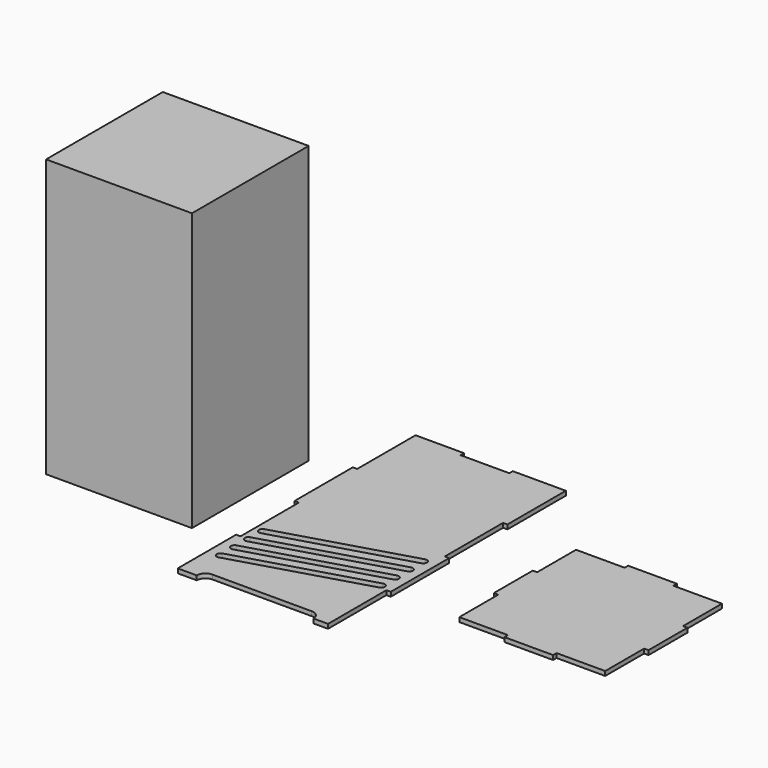
from build123d import *

# Parameters (mm, degrees)
F1_DEPTH = 3
F2_W     = 100
F2_H     = 100
F3_DEPTH = 190


# Not quite as in the source:
# - a feature names something its author has since deleted; it is built from what else it names


with BuildPart() as f1:
    # F0 (on Top) → F1 (new body)
    with BuildSketch(Plane.XY):
        with BuildLine():
            Line((-16.6666666667, 100), (-50, 100))
            Line((-50, 100), (-50, 50))
            Line((-50, 50), (-53, 50))
            Line((-53, 50), (-53, 0))
            Line((-53, 0), (-50, 0))
            Line((-50, 0), (-50, -50))
            Line((-50, -50), (-53, -50))
            Line((-53, -50), (-53, -100))
            Line((-53, -100), (-50, -100))
            Line((-50, -100), (-40, -100))
            ThreePointArc((-40, -100), (-38.2426406871, -95.7573593129), (-34, -94))
            Line((-34, -94), (34, -94))
            ThreePointArc((34, -94), (38.2426406871, -95.7573593129), (40, -100))
            Line((40, -100), (50, -100))
            Line((50, -100), (50, -50))
            Line((50, -50), (53, -50))
            Line((53, -50), (53, 0))
            Line((53, 0), (50, 0))
            Line((50, 0), (50, 50))
            Line((50, 50), (53, 50))
            Line((53, 50), (53, 100))
            Line((53, 100), (50, 100))
            Line((50, 100), (16.6666666667, 100))
            Line((16.6666666667, 100), (16.6666666667, 97))
            Line((16.6666666667, 97), (-16.6666666667, 97))
            Line((-16.6666666667, 97), (-16.6666666667, 100))
        make_face()
        with BuildLine():
            ThreePointArc((-43.7245756516, -76.3485534214), (-46.8767029852, -74.7472747846), (-45.2754243484, -71.595147451))
            Line((-45.2754243484, -71.595147451), (43.7885479556, -45.1109843029))
            ThreePointArc((43.7885479556, -45.1109843029), (46.8963350712, -46.7941332679), (45.2131861062, -49.9019203835))
            Line((45.2131861062, -49.9019203835), (-43.7245756516, -76.3485534214))
        make_face(mode=Mode.SUBTRACT)
        with BuildLine():
            Line((45.2131861062, -37.9019203835), (-43.7245756516, -64.3485534214))
            ThreePointArc((-43.7245756516, -64.3485534214), (-46.8767029852, -62.7472747846), (-45.2754243484, -59.595147451))
            Line((-45.2754243484, -59.595147451), (43.7885479556, -33.1109843029))
            ThreePointArc((43.7885479556, -33.1109843029), (46.8963350712, -34.7941332679), (45.2131861062, -37.9019203835))
        make_face(mode=Mode.SUBTRACT)
        with BuildLine():
            Line((45.2131861062, -25.9019203835), (-43.7245756516, -52.3485534214))
            ThreePointArc((-43.7245756516, -52.3485534214), (-46.8767029852, -50.7472747846), (-45.2754243484, -47.595147451))
            Line((-45.2754243484, -47.595147451), (43.7885479556, -21.1109843029))
            ThreePointArc((43.7885479556, -21.1109843029), (46.8963350712, -22.7941332679), (45.2131861062, -25.9019203835))
        make_face(mode=Mode.SUBTRACT)
        with BuildLine():
            Line((45.2131861062, -13.9019203835), (-43.7245756516, -40.3485534214))
            ThreePointArc((-43.7245756516, -40.3485534214), (-46.8767029852, -38.7472747846), (-45.2754243484, -35.595147451))
            Line((-45.2754243484, -35.595147451), (43.7885479556, -9.1109843029))
            ThreePointArc((43.7885479556, -9.1109843029), (46.8963350712, -10.7941332679), (45.2131861062, -13.9019203835))
        make_face(mode=Mode.SUBTRACT)
    extrude(amount=F1_DEPTH)


with BuildPart() as f1b:
    # F0 (on Top) → F1, piece 2 (new body)
    with BuildSketch(Plane.XY):
        Polygon((133.3333333333, 50), (100, 50), (100, 16.6666666667), (97, 16.6666666667), (97, -16.6666666667), (100, -16.6666666667), (100, -50), (133.3333333333, -50), (133.3333333333, -53), (166.6666666667, -53), (166.6666666667, -50), (200, -50), (200, -16.6666666667), (203, -16.6666666667), (203, 16.6666666667), (200, 16.6666666667), (200, 50), (166.6666666667, 50), (166.6666666667, 53), (133.3333333333, 53), align=None)
    extrude(amount=F1_DEPTH)


with BuildPart() as f3:
    # F2 (on Top) → F3 (new body)
    with BuildSketch(Plane.XY):
        with Locations((-129.7888755798, -4.3312566519)):
            Rectangle(F2_W, F2_H)
    extrude(amount=F3_DEPTH)


solid = Compound([f1.part, f1b.part, f3.part])
